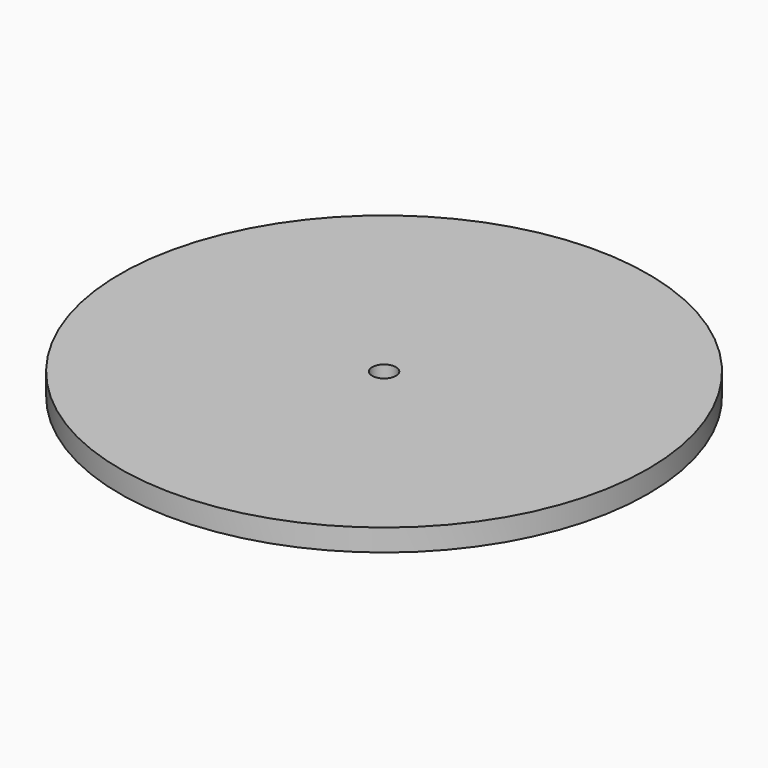
from build123d import *

# Parameters (mm, degrees)
F0_R     = 38.1
F1_DEPTH = 3.175
F2_R     = 1.7145
F3_DEPTH = 3.176


# Not quite as in the source:
# - a length typed as a fraction of an inch, garbled in the dataset ("3 / 203.2 mm" for 3/8 in), is restored


with BuildPart() as f1:
    # F0 (on Top) → F1 (new body)
    with BuildSketch(Plane.XY):
        Circle(F0_R)
    extrude(amount=F1_DEPTH)

    # F2 (on face) → F3 (cut, through all)
    with BuildSketch(Plane.XY.offset(3.175)):
        Circle(F2_R)
    extrude(amount=-F3_DEPTH, mode=Mode.SUBTRACT)


solid = f1.part
